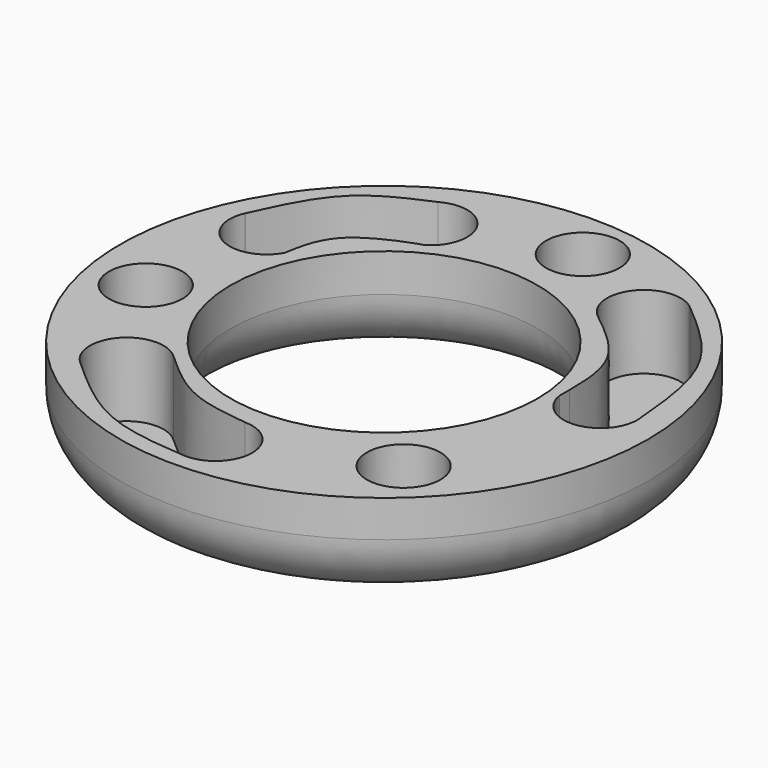
from build123d import *

# Parameters (mm, degrees)
F0_R     = 136.525
F0_R_2   = 79.375
F1_DEPTH = 50.8
F2_R     = 31.75
F4_R     = 19.05
F5_DEPTH = 38.1


# Not quite as in the source:
# - a fillet or chamfer that OpenCascade refuses, or shapes differently, is made with other operations: its cross-section is extruded or revolved along the edge and cut away or added


with BuildPart() as f1:
    # F0 (on Top) → F1 (new body)
    with BuildSketch(Plane.XY):
        with Locations((0, 2.0348737297)):
            Circle(F0_R)
        with Locations((0, 2.0348737297)):
            Circle(F0_R_2, mode=Mode.SUBTRACT)
    extrude(amount=F1_DEPTH)

    # F2
    f2_edges = [f1.edges().sort_by_distance(p)[0] for p in [
        (-136.525, 2.034874, 0),
    ]]
    fillet(f2_edges, radius=F2_R)

    # F3: fillet of radius 31.75 on 1 edges, made by hand

    # F3_s1 → F3_t2 (revolve, cut)
    with BuildSketch(Plane.XZ.offset(-2.0348737297)):
        with BuildLine():
            ThreePointArc((104.775, 0), (86.5315557516, 11.0280565913), (79.375, 31.1085197333))
            Line((79.375, 31.1085197333), (79.375, 0))
            Line((79.375, 0), (104.775, 0))
        make_face()
    revolve(axis=Axis((0, 2.0348737297, 0), (0, 0, 1)), mode=Mode.SUBTRACT)

    # F4 (on face) → F5 (cut)
    with BuildSketch(Plane.XY.offset(50.8)):
        with BuildLine():
            ThreePointArc((-83.5406207988, -89.6430518351), (-63.4036145785, -91.8975231455), (-52.6271930456, -74.7379660606))
            ThreePointArc((-52.6271930456, -74.7379660606), (-54.2244900151, -67.1021519632), (-58.7485218572, -60.74682739))
            ThreePointArc((-58.7485218572, -60.74682739), (-86.1351193385, -62.3334964102), (-83.5406207988, -89.6430518351))
        make_face()
        with BuildLine():
            ThreePointArc((-58.7485218572, -60.74682739), (-54.2244900151, -67.1021519632), (-52.6271930456, -74.7379660606))
            ThreePointArc((-52.6271930456, -74.7379660606), (-63.4036145785, -91.8975231455), (-83.5406207988, -89.6430518351))
            add(Edge.make_bspline(
                [(-2.8122035096, -125.8770781244), (-17.2926198403, -124.7913924318), (-47.475617869, -121.9892901593), (-71.1455318862, -100.7416006213), (-83.5406207988, -89.6430518351)],
                knots=[0.0299392112, 0.0299392112, 0.0299392112, 0.0299392112, 0.492539633, 1, 1, 1, 1], degree=3))
            ThreePointArc((-2.8122035096, -125.8770781244), (-18.9977495336, -105.6258243369), (0, -87.985793364))
            add(Edge.make_bspline(
                [(0, -87.985793364), (-10.8720074629, -86.6942500904), (-32.9218918222, -84.0821884123), (-50.0558702898, -68.5889761619), (-58.7485218572, -60.74682739)],
                knots=[0, 0, 0, 0, 0.493177557, 1, 1, 1, 1], degree=3))
        make_face()
        with BuildLine():
            ThreePointArc((19.05, -107.035793364), (13.4703841816, -93.5654091824), (0, -87.985793364))
            ThreePointArc((0, -87.985793364), (-18.9977495336, -105.6258243369), (-2.8122035096, -125.8770781244))
            add(Edge.make_bspline(
                [(0, -126.085793364), (-0.9375128174, -126.0165583722), (-1.8750399814, -125.9473430264), (-2.8122035096, -125.8770781244)],
                knots=[0, 0, 0, 0, 0.0299392112, 0.0299392112, 0.0299392112, 0.0299392112], degree=3))
            ThreePointArc((0, -126.085793364), (13.4703841816, -120.5061775457), (19.05, -107.035793364))
        make_face()
        with Locations((74.0118548274, -77.8447389603)):
            Circle(F4_R)
        with BuildLine():
            add(Edge.make_bspline(
                [(78.9350842893, 101.6695168607), (78.0894264406, 102.3824779177), (77.2423258351, 103.0946725571), (76.3952137559, 103.80686703)],
                knots=[0.9690492423, 0.9690492423, 0.9690492423, 0.9690492423, 1, 1, 1, 1], degree=3))
            ThreePointArc((76.3952137559, 103.80686703), (50.1528602496, 99.5766504715), (53.6856126427, 73.2313376017))
            ThreePointArc((53.6856126427, 73.2313376017), (73.7786820966, 71.0869181488), (84.4960042715, 88.2178544998))
            ThreePointArc((84.4960042715, 88.2178544998), (83.0509676958, 95.4957499944), (78.9350842893, 101.6695168607))
        make_face()
        with BuildLine():
            ThreePointArc((84.4960042715, 88.2178544998), (73.7786820966, 71.0869181488), (53.6856126427, 73.2313376017))
            add(Edge.make_bspline(
                [(84.7416844545, 15.995532865), (84.7371406471, 26.5933171928), (83.3814622914, 49.6305752088), (64.2349565752, 64.8357897445), (53.6856126427, 73.2313376017)],
                knots=[0.0840841786, 0.0840841786, 0.0840841786, 0.0840841786, 0.4948689966, 1, 1, 1, 1], degree=3))
            ThreePointArc((84.7416844545, 15.995532865), (103.773764442, 31.641700355), (122.3236967579, 15.4268109984))
            add(Edge.make_bspline(
                [(122.3236967579, 15.4268109984), (120.6881998826, 33.4274356769), (117.5065684963, 68.2125390548), (91.7120360038, 90.8974664243), (78.9350842893, 101.6695168607)],
                knots=[0, 0, 0, 0, 0.5014176382, 0.9690492423, 0.9690492423, 0.9690492423, 0.9690492423], degree=3))
            ThreePointArc((78.9350842893, 101.6695168607), (83.0509676958, 95.4957499944), (84.4960042715, 88.2178544998))
        make_face()
        with BuildLine():
            ThreePointArc((122.3236967579, 15.4268109984), (103.773764442, 31.641700355), (84.7416844545, 15.995532865))
            add(Edge.make_bspline(
                [(84.6941362488, 9.4655427217), (84.7182599274, 11.6458483909), (84.7426145335, 13.8262560296), (84.7416844545, 15.995532865)],
                knots=[0, 0, 0, 0, 0.0840841786, 0.0840841786, 0.0840841786, 0.0840841786], degree=3))
            ThreePointArc((84.6941362488, 9.4655427217), (105.0550223499, -6.3913539202), (122.5355172038, 12.5938812271))
            ThreePointArc((122.5355172038, 12.5938812271), (122.4824882848, 14.0143000905), (122.3236967579, 15.4268109984))
        make_face()
        with Locations((-106.1858087778, -19.3491019309)):
            Circle(F4_R)
        with Locations((14.8240327835, 111.9937822223)):
            Circle(F4_R)
        with BuildLine():
            add(Edge.make_bspline(
                [(-114.1068806006, 54.731659933), (-114.0705377389, 54.8113823903), (-114.0341951825, 54.8911049607), (-113.9978523202, 54.9708268217)],
                knots=[0, 0, 0, 0, 0.0029673982, 0.0029673982, 0.0029673982, 0.0029673982], degree=3))
            ThreePointArc((-114.1068806006, 54.731659933), (-105.2006835176, 29.8918835009), (-80.0197694208, 37.7821563054))
            add(Edge.make_bspline(
                [(-80.0197694208, 37.7821563054), (-79.3943245384, 41.4243222007), (-78.7675270407, 45.0666971781), (-77.740869501, 48.6034247835)],
                knots=[0, 0, 0, 0, 0.1730413551, 0.1730413551, 0.1730413551, 0.1730413551], degree=3))
            ThreePointArc((-77.740869501, 48.6034247835), (-93.4238298796, 65.7123618791), (-113.9978523202, 54.9708268217))
        make_face()
        with BuildLine():
            add(Edge.make_bspline(
                [(-113.9978523202, 54.9708268217), (-107.6814847314, 68.8264382664), (-95.452579475, 95.5712033941), (-71.1959439676, 106.0972459264), (-59.4868722066, 111.1759600983)],
                knots=[0.0029673982, 0.0029673982, 0.0029673982, 0.0029673982, 0.5186994147, 1, 1, 1, 1], degree=3))
            ThreePointArc((-113.9978523202, 54.9708268217), (-93.4238298796, 65.7123618791), (-77.740869501, 48.6034247835))
            add(Edge.make_bspline(
                [(-77.740869501, 48.6034247835), (-76.0045089103, 54.5850050058), (-70.5050739876, 65.4294674019), (-53.8065169404, 73.305008588), (-47.9266097256, 75.67092688)],
                knots=[0.1730413551, 0.1730413551, 0.1730413551, 0.1730413551, 0.4657019337, 0.7318600546, 0.7318600546, 0.7318600546, 0.7318600546], degree=3))
            ThreePointArc((-47.9266097256, 75.67092688), (-68.2199127162, 88.6980268466), (-59.4868722066, 111.1759600983))
        make_face()
        with BuildLine():
            ThreePointArc((-31.0558846712, 94.5958644152), (-40.5091485737, 111.0520230275), (-59.4868722066, 111.1759600983))
            ThreePointArc((-59.4868722066, 111.1759600983), (-68.2199127162, 88.6980268466), (-47.9266097256, 75.67092688))
            add(Edge.make_bspline(
                [(-47.9266097256, 75.67092688), (-43.5392758956, 77.4362733357), (-40.3063077929, 78.4304649494), (-40.1444315528, 78.3578857303)],
                knots=[0.7318600546, 0.7318600546, 0.7318600546, 0.7318600546, 0.9304557952, 0.9304557952, 0.9304557952, 0.9304557952], degree=3))
            ThreePointArc((-40.1444315528, 78.3578857303), (-33.4825850303, 85.29164983), (-31.0558846712, 94.5958644152))
        make_face()
    extrude(amount=-F5_DEPTH, mode=Mode.SUBTRACT)


solid = f1.part
